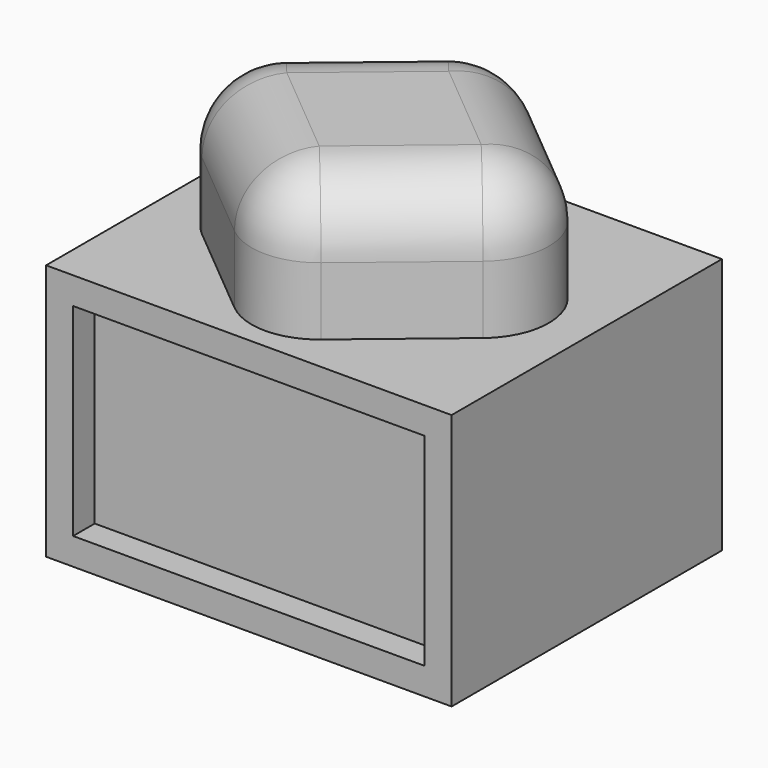
from build123d import *

# Parameters (mm, degrees)
F0_W     = 30
F0_H     = 18.981232
F1_DEPTH = 12.5
F3_DEPTH = 10
F4_R     = 5
F6_DEPTH = 2


with BuildPart() as f1:
    # F0 (on Front) → F1 (new body, symmetric)
    with BuildSketch(Plane.XZ):
        with Locations((15, 9.490616)):
            Rectangle(F0_W, F0_H)
    extrude(amount=F1_DEPTH, both=True)

    # F2 (on face) → F3 (join)
    with BuildSketch(Plane.XY.offset(18.981232)):
        Polygon((15, 12.5), (0, 0), (15, -12.5), (30, 0), align=None)
    extrude(amount=F3_DEPTH)

    # F4
    f4_edges = [f1.edges().sort_by_distance(p)[0] for p in [
        (7.5, 6.25, 28.981232),
        (7.5, -6.25, 28.981232),
        (22.5, -6.25, 28.981232),
        (22.5, 6.25, 28.981232),
        (15, -12.5, 23.981232),
        (30, 0, 23.981232),
        (15, 12.5, 23.981232),
        (0, 0, 23.981232),
    ]]
    fillet(f4_edges, radius=F4_R)

    # F5 (on face) → F6 (cut)
    with BuildSketch(Plane.XZ.offset(12.5)):
        Polygon((15, 16.981232), (2, 16.981232), (2, 2), (28, 2), (28, 16.981232), align=None)
    extrude(amount=-F6_DEPTH, mode=Mode.SUBTRACT)


solid = f1.part
